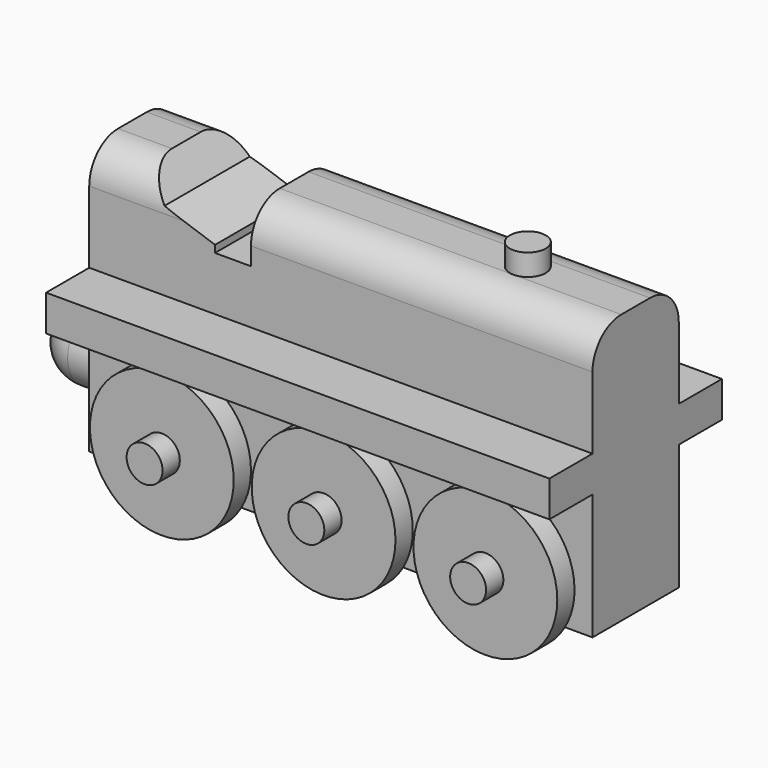
from build123d import *

# Parameters (mm, degrees)
F0_W      = 70
F0_H      = 15
F1_DEPTH  = 8.75
F2_W      = 70
F2_H      = 30
F3_DEPTH  = 5
F4_W      = 70
F4_H      = 15
F5_DEPTH  = 15
F6_W      = 5
F6_H      = 5
F8_R      = 10
F9_DEPTH  = 3
F10_R     = 10
F11_DEPTH = 3
F12_R     = 10
F13_DEPTH = 3
F14_R     = 2.5
F15_DEPTH = 3
F16_R     = 2.5
F17_DEPTH = 3
F18_R     = 2.5
F19_DEPTH = 3
F20_R     = 2.5
F21_DEPTH = 3
F23_DEPTH = 15
F24_R     = 5
F25_R     = 5


# Not quite as in the source:
# - a pattern or mirror of a feature is missing from the dataset's text; its kind, count and spacing are read off the source's solid


with BuildPart() as f1:
    # F0 (on Top) → F1 (new body, symmetric)
    with BuildSketch(Plane.XY):
        Rectangle(F0_W, F0_H)
    extrude(amount=F1_DEPTH, both=True)

    # F2 (on face) → F3 (join)
    with BuildSketch(Plane.XY.offset(8.75)):
        Rectangle(F2_W, F2_H)
    extrude(amount=F3_DEPTH)

    # F4 (on face) → F5 (join)
    with BuildSketch(Plane.XY.offset(13.75)):
        Rectangle(F4_W, F4_H)
    extrude(amount=F5_DEPTH)

    # F6 (on Front) → F7 (revolve)
    with BuildSketch(Plane.XZ):
        with Locations((-37.5, -2.5)):
            Rectangle(F6_W, F6_H)
    revolve(axis=Axis((0.3605282434, 0, 0), (1, 0, 0)))

    # F8 (on face) → F9 (join)
    with BuildSketch(Plane.XZ.offset(7.5)):
        with Locations((-22.5, -3.75)):
            Circle(F8_R)
    f9 = extrude(amount=F9_DEPTH)

    # F9_copies: F9 across plane
    add(f9.mirror(Plane.ZX))

    # F10 (on face) → F11 (join)
    with BuildSketch(Plane.XZ.offset(7.5)):
        with Locations((0, -3.75)):
            Circle(F10_R)
    f11 = extrude(amount=F11_DEPTH)

    # F11_copies: F11 across plane
    add(f11.mirror(Plane.ZX))

    # F12 (on face) → F13 (join)
    with BuildSketch(Plane.XZ.offset(7.5)):
        with Locations((22.5, -3.75)):
            Circle(F12_R)
    f13 = extrude(amount=F13_DEPTH)

    # F13_copies: F13 across plane
    add(f13.mirror(Plane.ZX))

    # F14 (on face) → F15 (join)
    with BuildSketch(Plane.XZ.offset(10.5)):
        with Locations((-22.5, -3.75)):
            Circle(F14_R)
    f15 = extrude(amount=F15_DEPTH)

    # F15_copies: F15 across plane
    add(f15.mirror(Plane.ZX))

    # F16 (on face) → F17 (join)
    with BuildSketch(Plane.XZ.offset(10.5)):
        with Locations((0, -3.75)):
            Circle(F16_R)
    f17 = extrude(amount=F17_DEPTH)

    # F17_copies: F17 across plane
    add(f17.mirror(Plane.ZX))

    # F18 (on face) → F19 (join)
    with BuildSketch(Plane.XZ.offset(10.5)):
        with Locations((22.5, -3.75)):
            Circle(F18_R)
    f19 = extrude(amount=F19_DEPTH)

    # F19_copies: F19 across plane
    add(f19.mirror(Plane.ZX))

    # F20 (on face) → F21 (join)
    with BuildSketch(Plane.XY.offset(28.75)):
        with Locations((20, 0)):
            Circle(F20_R)
    extrude(amount=F21_DEPTH)

    # F22 (on face) → F23 (cut, through all)
    with BuildSketch(Plane.XZ.offset(7.5)):
        Polygon((-12.5, 28.75), (-27.5, 28.75), (-24.5953480316, 24.6802337976), (-17.5, 22.25), (-17.5, 21.25), (-12.5, 21.25), align=None)
    extrude(amount=-F23_DEPTH, mode=Mode.SUBTRACT)

    # F24
    f24_edges = [f1.edges().sort_by_distance(p)[0] for p in [
        (11.25, -7.5, 28.75),
        (11.25, 7.5, 28.75),
    ]]
    fillet(f24_edges, radius=F24_R)

    # F25
    f25_edges = [f1.edges().sort_by_distance(p)[0] for p in [
        (-31.25, -7.5, 28.75),
        (-31.25, 7.5, 28.75),
    ]]
    fillet(f25_edges, radius=F25_R)

    # F26 (on Front) → F27 (revolve)
    with BuildSketch(Plane.XZ):
        with BuildLine():
            Line((-40, 0), (-40, 5))
            ThreePointArc((-40, 5), (-43.5355339059, 3.5355339059), (-45, 0))
            Line((-45, 0), (-40, 0))
        make_face()
    revolve(axis=Axis((-36.5614034235, 0, 0), (1, 0, 0)))


solid = f1.part
